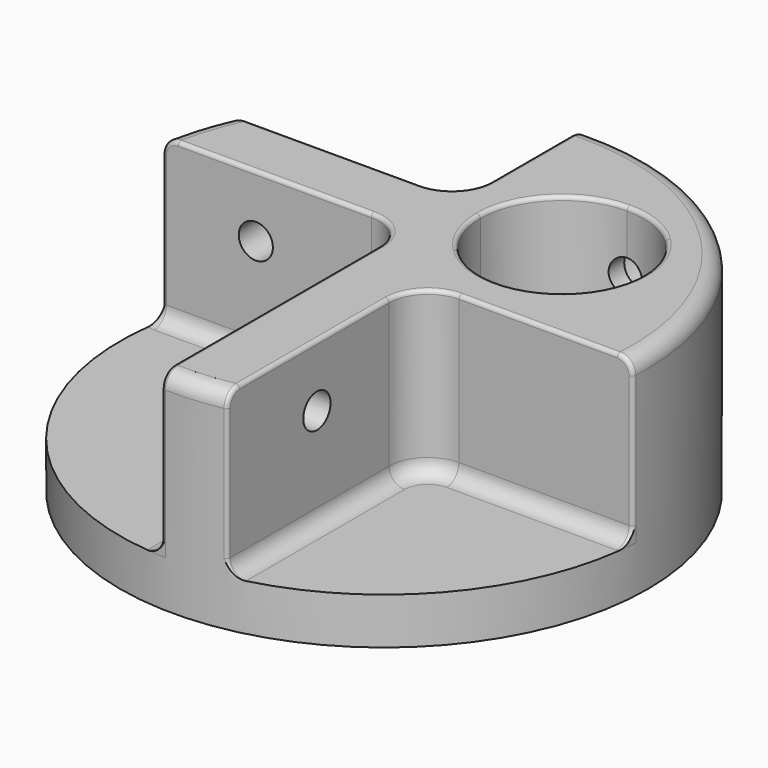
from build123d import *

# Parameters (mm, degrees)
F0_R            = 34
F1_DEPTH        = 27
F3_R            = 2
F4_DEPTH        = 21
F5_R            = 0.5
F6_R            = 5
F7_DEPTH        = 7
F9_D            = 4.4
F9_DEPTH        = 10
F9_TIP          = 1.3218933619
F11_D           = 4.4
F11_DEPTH       = 10
F11_TIP         = 1.3218933619
F14_D           = 4.4
F14_DEPTH       = 26
F14_START       = 4.9876232
F14_CBORE_D     = 10
F14_CBORE_DEPTH = 3.5
F14_TIP         = 1.3218933619
F19_T1_DEPTH    = 21.9087906991
F19_T3_DEPTH    = 34.5176143137
F19_T5_DEPTH    = 26.396371076
F19_T7_DEPTH    = 14.4548261445
F19_T10_ANGLE   = 90
F19_T14_DEPTH   = 25.5859128064
F19_S15_R       = 34
F19_T16_DEPTH   = 14
F19_T18_ANGLE   = 90
F19_T22_DEPTH   = 24.1848193523
F19_S23_R       = 34
F19_T24_DEPTH   = 14
F19_T26_ANGLE   = 90
F19_T30_ANGLE   = 359.64
F19_S31_R       = 34
F19_T32_DEPTH   = 6
F19_T36_ANGLE   = 359.64
F19_S37_R       = 34
F19_T38_DEPTH   = 8
F19_T42_ANGLE   = 359.64
F19_S43_R       = 34
F19_T44_DEPTH   = 6
F19_T48_ANGLE   = 359.64
F19_S49_R       = 34
F19_T50_DEPTH   = 8
F19_T54_ANGLE   = 359.64
F19_S55_R       = 34
F19_T56_DEPTH   = 8
F19_T60_ANGLE   = 359.64
F19_S61_R       = 34
F19_T62_DEPTH   = 8


# Not quite as in the source:
# - a fillet or chamfer that OpenCascade refuses, or shapes differently, is made with other operations: its cross-section is extruded or revolved along the edge and cut away or added


with BuildPart() as f1:
    # F0 (on Top) → F1 (new body)
    with BuildSketch(Plane.XY):
        Circle(F0_R)
    extrude(amount=F1_DEPTH)

    # F3
    f3_edges = [f1.edges().sort_by_distance(p)[0] for p in [
        (-34, 0, 27),
    ]]
    fillet(f3_edges, radius=F3_R)

    # F2 (on face) → F4 (cut)
    with BuildSketch(Plane.XY.offset(27)):
        with BuildLine():
            ThreePointArc((-1.4607573942, 33.9686059154), (-19.0343409004, 28.1725729476), (-30.9696622526, 14.0313940846))
            Line((-30.9696622526, 14.0313940846), (-6.4607573942, 14.0313940846))
            ThreePointArc((-6.4607573942, 14.0313940846), (-2.9252234883, 15.4958601787), (-1.4607573942, 19.0313940846))
            Line((-1.4607573942, 19.0313940846), (-1.4607573942, 33.9686059154))
        make_face()
        with BuildLine():
            Line((-6.4607573942, 6.0313940846), (-33.4607573942, 6.0313940846))
            ThreePointArc((-33.4607573942, 6.0313940846), (-26.5495395211, -21.2396316169), (-1.4607573942, -33.9686059154))
            Line((-1.4607573942, -33.9686059154), (-1.4607573942, 1.0313940846))
            ThreePointArc((-1.4607573942, 1.0313940846), (-2.9252234883, 4.5669279905), (-6.4607573942, 6.0313940846))
        make_face()
        with BuildLine():
            Line((6.5392426058, -7.3652260017), (6.5392426058, -33.3652260017))
            ThreePointArc((6.5392426058, -33.3652260017), (25.4841060164, -22.5068953999), (33.9176311962, -2.3652260017))
            Line((33.9176311962, -2.3652260017), (11.5392426058, -2.3652260017))
            ThreePointArc((11.5392426058, -2.3652260017), (8.0037086998, -3.8296920957), (6.5392426058, -7.3652260017))
        make_face()
        with BuildLine():
            Line((12.7279220614, 12.7279220614), (12.7279220614, 23.2279220614))
            ThreePointArc((12.7279220614, 23.2279220614), (5.3033008589, 20.1525432638), (2.2279220614, 12.7279220614))
            ThreePointArc((2.2279220614, 12.7279220614), (3.02718697, 8.7097460215), (5.3033008589, 5.3033008589))
            Line((5.3033008589, 5.3033008589), (12.7279220614, 12.7279220614))
        make_face()
        with BuildLine():
            ThreePointArc((23.2279220614, 12.7279220614), (22.4286571527, 16.7460981012), (20.1525432638, 20.1525432638))
            Line((20.1525432638, 20.1525432638), (12.7279220614, 12.7279220614))
            Line((12.7279220614, 12.7279220614), (5.3033008589, 5.3033008589))
            ThreePointArc((5.3033008589, 5.3033008589), (16.7460981012, 3.02718697), (23.2279220614, 12.7279220614))
        make_face()
        with BuildLine():
            ThreePointArc((20.1525432638, 20.1525432638), (16.7460981012, 22.4286571527), (12.7279220614, 23.2279220614))
            Line((12.7279220614, 23.2279220614), (12.7279220614, 12.7279220614))
            Line((12.7279220614, 12.7279220614), (20.1525432638, 20.1525432638))
        make_face()
    extrude(amount=-F4_DEPTH, mode=Mode.SUBTRACT)

    # F5
    f5_edges = [f1.edges().sort_by_distance(p)[0] for p in [
        (5.303301, 5.303301, 27),
        (21.725856, -2.365226, 27),
        (22.9455, 22.304798, 27),
        (-1.460757, 25.499018, 27),
        (-2.925223, 15.49586, 27),
        (-17.610226, 14.031394, 27),
        (-30.357754, 10.119623, 27),
        (-18.943608, 6.031394, 27),
        (-2.925223, 4.566928, 27),
        (-1.460757, -15.467624, 27),
        (2.559447, -31.89748, 27),
        (6.539243, -19.344975, 27),
        (8.003709, -3.829692, 27),
        (33.917631, -2.365226, 15.5),
        (6.539243, -33.365226, 15.5),
        (-1.460757, -33.968606, 15.5),
        (-33.460757, 6.031394, 15.5),
        (-30.969662, 14.031394, 15.5),
        (-1.460757, 33.968606, 15.5),
        (-1.460757, 33.381967, 26.414515),
        (-30.291874, 14.031394, 26.443993),
        (-32.86023, 6.031394, 26.419242),
        (-1.460757, -33.381967, 26.414515),
        (6.539243, -32.762022, 26.420143),
        (33.329624, -2.365226, 26.414985),
    ]]
    fillet(f5_edges, radius=F5_R)

    # F6 (on face) → F7 (cut)
    with BuildSketch(Plane(origin=(0, 0, 0), x_dir=(1, 0, 0), z_dir=(0, 0, -1))):
        with Locations((12.7206174657, -12.7342063934)):
            Circle(F6_R)
    extrude(amount=-F7_DEPTH, mode=Mode.SUBTRACT)

    # F9
    with Locations(Plane(origin=(-1.4607573942, 0, 0), x_dir=(0, -1, 0), z_dir=(-1, 0, 0))):
        with Locations((18.9860145608, 19)):
            Hole(F9_D / 2, depth=F9_DEPTH)
            with Locations((0, 0, -(F9_DEPTH + F9_TIP / 2))):  # 118° drill point
                Cone(0, F9_D / 2, F9_TIP, mode=Mode.SUBTRACT)

    # F11
    with Locations(Plane.XZ.offset(-6.0313940846)):
        with Locations((-21.3475333728, 19)):
            Hole(F11_D / 2, depth=F11_DEPTH)
            with Locations((0, 0, -(F11_DEPTH + F11_TIP / 2))):  # 118° drill point
                Cone(0, F11_D / 2, F11_TIP, mode=Mode.SUBTRACT)

    # F14
    # its depths count from where the whole tool has entered the part; down to there all is cleared
    with Locations(Plane(origin=(0, 34, 0), x_dir=(1, 0, 0), z_dir=(0, 1, 0)).offset(-F14_START)):
        with Locations((12.728, -19)):
            CounterBoreHole(F14_D / 2, F14_CBORE_D / 2, F14_CBORE_DEPTH, depth=F14_DEPTH)
            with Locations((0, 0, -(F14_DEPTH + F14_TIP / 2))):  # 118° drill point
                Cone(0, F14_D / 2, F14_TIP, mode=Mode.SUBTRACT)


with BuildPart() as f15_1:
    # F15: copy of F1
    add(f1.part)


with BuildPart() as f16_1:
    # F16: copy of F1
    add(f1.part)


with BuildPart() as f1_1:
    add(f1.part)

    # F19: fillet of radius 2 on 9 edges, made by hand

    # F19_s2 → F19_t1 (join)
    with BuildSketch(Plane.YZ.offset(11.5392426058)):
        with BuildLine():
            ThreePointArc((-4.3652260017, 6), (-2.9510124393, 6.5857864376), (-2.3652260017, 8))
            Line((-2.3652260017, 8), (-2.3652260017, 6))
            Line((-2.3652260017, 6), (-4.3652260017, 6))
        make_face()
    extrude(amount=F19_T1_DEPTH)

    # F19_s4 → F19_t3 (join)
    with BuildSketch(Plane.XZ.offset(-1.0313940846)):
        with BuildLine():
            ThreePointArc((-3.4607573942, 6), (-2.0465438319, 6.5857864376), (-1.4607573942, 8))
            Line((-1.4607573942, 8), (-1.4607573942, 6))
            Line((-1.4607573942, 6), (-3.4607573942, 6))
        make_face()
    extrude(amount=F19_T3_DEPTH)

    # F19_s6 → F19_t5 (join)
    with BuildSketch(Plane.YZ.offset(-32.8571284703)):
        with BuildLine():
            ThreePointArc((4.0313940846, 6), (5.445607647, 6.5857864376), (6.0313940846, 8))
            Line((6.0313940846, 8), (6.0313940846, 6))
            Line((6.0313940846, 6), (4.0313940846, 6))
        make_face()
    extrude(amount=F19_T5_DEPTH)

    # F19_s8 → F19_t7 (join)
    with BuildSketch(Plane.XZ.offset(-33.4862202291)):
        with BuildLine():
            ThreePointArc((-3.4607573942, 6), (-2.0465438319, 6.5857864376), (-1.4607573942, 8))
            Line((-1.4607573942, 8), (-1.4607573942, 6))
            Line((-1.4607573942, 6), (-3.4607573942, 6))
        make_face()
    extrude(amount=F19_T7_DEPTH)

    # F19_s9 → F19_t10 (revolve)
    with BuildSketch(Plane.YZ.offset(11.5392426058)):
        with BuildLine():
            ThreePointArc((-4.3652260017, 6), (-2.9510124393, 6.5857864376), (-2.3652260017, 8))
            Line((-2.3652260017, 8), (-2.3652260017, 6))
            Line((-2.3652260017, 6), (-4.3652260017, 6))
        make_face()
    revolve(axis=Axis((11.5392426058, -7.3652260017, 6), (0, 0, 1)), revolution_arc=F19_T10_ANGLE)


with BuildPart() as f19_tool12:
    # F19_s13 → F19_t14 (new body)
    with BuildSketch(Plane.XZ.offset(7.3652260017)):
        with BuildLine():
            ThreePointArc((8.5392426058, 6), (7.1250290434, 6.5857864376), (6.5392426058, 8))
            Line((6.5392426058, 8), (6.5392426058, 6))
            Line((6.5392426058, 6), (8.5392426058, 6))
        make_face()
    extrude(amount=F19_T14_DEPTH)

    # F19_s15 → F19_t16 (intersect, symmetric)
    with BuildSketch(Plane.XY.offset(7)):
        Circle(F19_S15_R)
    extrude(amount=F19_T16_DEPTH, both=True, mode=Mode.INTERSECT)


with BuildPart() as f1_2:
    add(f1_1.part)

    # F19_t11: union F19_tool12
    add(f19_tool12.part)

    # F19_s17 → F19_t18 (revolve)
    with BuildSketch(Plane.XZ.offset(-1.0313940846)):
        with BuildLine():
            ThreePointArc((-3.4607573942, 6), (-2.0465438319, 6.5857864376), (-1.4607573942, 8))
            Line((-1.4607573942, 8), (-1.4607573942, 6))
            Line((-1.4607573942, 6), (-3.4607573942, 6))
        make_face()
    revolve(axis=Axis((-6.4607573942, 1.0313940846, 6), (0, 0, 1)), revolution_arc=F19_T18_ANGLE)


with BuildPart() as f19_tool20:
    # F19_s21 → F19_t22 (new body)
    with BuildSketch(Plane.YZ.offset(-30.6455767465)):
        with BuildLine():
            ThreePointArc((16.0313940846, 6), (14.6171805222, 6.5857864376), (14.0313940846, 8))
            Line((14.0313940846, 8), (14.0313940846, 6))
            Line((14.0313940846, 6), (16.0313940846, 6))
        make_face()
    extrude(amount=F19_T22_DEPTH)

    # F19_s23 → F19_t24 (intersect, symmetric)
    with BuildSketch(Plane.XY.offset(7)):
        Circle(F19_S23_R)
    extrude(amount=F19_T24_DEPTH, both=True, mode=Mode.INTERSECT)


with BuildPart() as f1_3:
    add(f1_2.part)

    # F19_t19: union F19_tool20
    add(f19_tool20.part)

    # F19_s25 → F19_t26 (revolve)
    with BuildSketch(Plane.YZ.offset(-6.4607573942)):
        with BuildLine():
            ThreePointArc((16.0313940846, 6), (14.6171805222, 6.5857864376), (14.0313940846, 8))
            Line((14.0313940846, 8), (14.0313940846, 6))
            Line((14.0313940846, 6), (16.0313940846, 6))
        make_face()
    revolve(axis=Axis((-6.4607573942, 19.0313940846, 6), (0, 0, 1)), revolution_arc=F19_T26_ANGLE)


with BuildPart() as f19_tool28:
    # F19_s29 → F19_t30 (revolve)
    with BuildSketch(Plane.XZ.offset(-33.4862202291)):
        with BuildLine():
            ThreePointArc((-3.4607573942, 6), (-2.0465438319, 6.5857864376), (-1.4607573942, 8))
            Line((-1.4607573942, 8), (-1.4607573942, 6))
            Line((-1.4607573942, 6), (-3.4607573942, 6))
        make_face()
    revolve(axis=Axis((-0.9607573942, 33.4862202291, 6), (0, 0, -1)), revolution_arc=F19_T30_ANGLE)

    # F19_s31 → F19_t32 (intersect, symmetric)
    with BuildSketch(Plane.XY.offset(7.7)):
        Circle(F19_S31_R)
    extrude(amount=F19_T32_DEPTH, both=True, mode=Mode.INTERSECT)


with BuildPart() as f1_4:
    add(f1_3.part)

    # F19_t27: union F19_tool28
    add(f19_tool28.part)


with BuildPart() as f19_tool34:
    # F19_s35 → F19_t36 (revolve)
    with BuildSketch(Plane.YZ.offset(-30.6455767465)):
        with BuildLine():
            ThreePointArc((14.0313940846, 8), (14.6171805222, 6.5857864376), (16.0313940846, 6))
            Line((16.0313940846, 6), (14.0313940846, 6))
            Line((14.0313940846, 6), (14.0313940846, 8))
        make_face()
    revolve(axis=Axis((-30.6455767465, 13.5313940846, 6), (0, 0, 1)), revolution_arc=F19_T36_ANGLE)

    # F19_s37 → F19_t38 (intersect, symmetric)
    with BuildSketch(Plane.XY.offset(7)):
        Circle(F19_S37_R)
    extrude(amount=F19_T38_DEPTH, both=True, mode=Mode.INTERSECT)


with BuildPart() as f1_5:
    add(f1_4.part)

    # F19_t33: union F19_tool34
    add(f19_tool34.part)


with BuildPart() as f19_tool40:
    # F19_s41 → F19_t42 (revolve)
    with BuildSketch(Plane(origin=(-32.8147944606, -0.2061841477, 0), x_dir=(0, 0, 1), z_dir=(-0.9999802609, -0.006283144, 0))):
        with BuildLine():
            ThreePointArc((6, 4.237711229), (6.5857864376, 5.6519247913), (8, 6.237711229))
            Line((8, 6.237711229), (6, 6.237711229))
            Line((6, 6.237711229), (6, 4.237711229))
        make_face()
    revolve(axis=Axis((-32.8571284703, 6.5313940846, 6), (0, 0, 1)), revolution_arc=F19_T42_ANGLE)

    # F19_s43 → F19_t44 (intersect, symmetric)
    with BuildSketch(Plane.XY.offset(7.7)):
        Circle(F19_S43_R)
    extrude(amount=F19_T44_DEPTH, both=True, mode=Mode.INTERSECT)


with BuildPart() as f1_6:
    add(f1_5.part)

    # F19_t39: union F19_tool40
    add(f19_tool40.part)


with BuildPart() as f19_tool46:
    # F19_s47 → F19_t48 (revolve)
    with BuildSketch(Plane(origin=(-0.2104325182, -33.4909347213, 0), x_dir=(0, 0, 1), z_dir=(-0.006283144, -0.9999802609, 0))):
        with BuildLine():
            ThreePointArc((8, 1.2503396871), (6.5857864376, 1.8361261248), (6, 3.2503396871))
            Line((6, 3.2503396871), (6, 1.2503396871))
            Line((6, 1.2503396871), (8, 1.2503396871))
        make_face()
    revolve(axis=Axis((-0.9607573942, -33.4862202291, 6), (0, 0, -1)), revolution_arc=F19_T48_ANGLE)

    # F19_s49 → F19_t50 (intersect, symmetric)
    with BuildSketch(Plane.XY.offset(7)):
        Circle(F19_S49_R)
    extrude(amount=F19_T50_DEPTH, both=True, mode=Mode.INTERSECT)


with BuildPart() as f1_7:
    add(f1_6.part)

    # F19_t45: union F19_tool46
    add(f19_tool46.part)


with BuildPart() as f19_tool52:
    # F19_s53 → F19_t54 (revolve)
    with BuildSketch(Plane(origin=(0.2072710788, -32.9877826481, 0), x_dir=(0, 0, 1), z_dir=(0.006283144, -0.9999802609, 0))):
        with BuildLine():
            ThreePointArc((6, -8.3320866473), (6.5857864376, -6.9178730849), (8, -6.3320866473))
            Line((8, -6.3320866473), (6, -6.3320866473))
            Line((6, -6.3320866473), (6, -8.3320866473))
        make_face()
    revolve(axis=Axis((6.0392426058, -32.9511388081, 6), (0, 0, 1)), revolution_arc=F19_T54_ANGLE)

    # F19_s55 → F19_t56 (intersect, symmetric)
    with BuildSketch(Plane.XY.offset(7.7)):
        Circle(F19_S55_R)
    extrude(amount=F19_T56_DEPTH, both=True, mode=Mode.INTERSECT)


with BuildPart() as f1_8:
    add(f1_7.part)

    # F19_t51: union F19_tool52
    add(f19_tool52.part)


with BuildPart() as f19_tool58:
    # F19_s59 → F19_t60 (revolve)
    with BuildSketch(Plane(origin=(33.458432099, -0.2102282955, 0), x_dir=(0, 0, 1), z_dir=(0.9999802609, -0.006283144, 0))):
        with BuildLine():
            ThreePointArc((8, 2.1550303751), (6.5857864376, 2.7408168127), (6, 4.1550303751))
            Line((6, 4.1550303751), (6, 2.1550303751))
            Line((6, 2.1550303751), (8, 2.1550303751))
        make_face()
    revolve(axis=Axis((33.4480333049, -1.8652260017, 6), (0, 0, -1)), revolution_arc=F19_T60_ANGLE)

    # F19_s61 → F19_t62 (intersect, symmetric)
    with BuildSketch(Plane.XY.offset(7)):
        Circle(F19_S61_R)
    extrude(amount=F19_T62_DEPTH, both=True, mode=Mode.INTERSECT)


with BuildPart() as f1_9:
    add(f1_8.part)

    # F19_t57: union F19_tool58
    add(f19_tool58.part)


solid = f1_9.part
